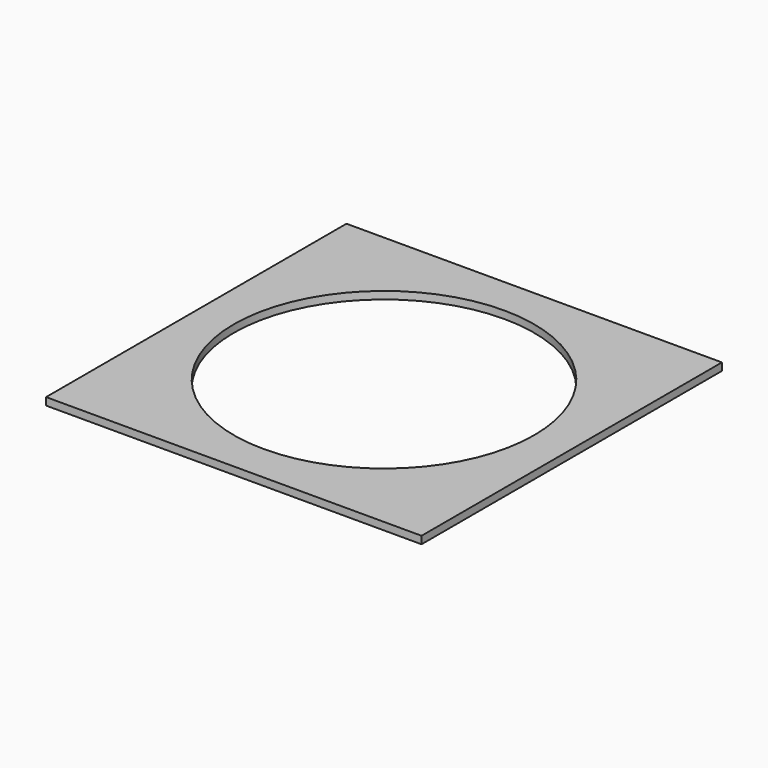
from build123d import *

# Parameters (mm, degrees)
F0_W     = 127
F0_H     = 127
F1_DEPTH = 2.54
F4_D     = 101.6


# Not quite as in the source:
# - the program builds the solid bodies; features that only make, move or delete a surface that nothing else refers to are left out


with BuildPart() as f1:
    # F0 (on Top) → F1 (new body)
    with BuildSketch(Plane.XY):
        Rectangle(F0_W, F0_H)
    extrude(amount=F1_DEPTH)

    # F4 (through all)
    with Locations(Plane(origin=(0, 0, 0), x_dir=(1, 0, 0), z_dir=(0, 0, -1))):
        with Locations((0, 0)):
            Hole(F4_D / 2)


solid = f1.part
